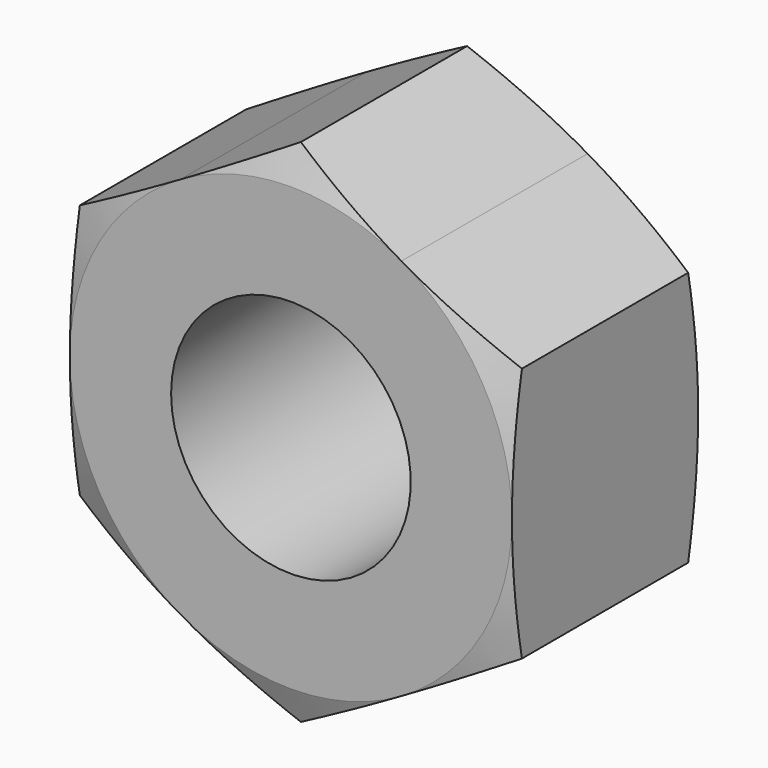
from build123d import *

# Parameters (mm, degrees)
F3_DEPTH      = 38
F3_DEPTH_BACK = 10.001
F4_D          = 10.3


# Not quite as in the source:
# - an extrude ends at something that could not be found from the text; its depth is read off the source's solid


with BuildPart() as f2:
    # F1 (on Right) → F2 (revolve)
    with BuildSketch(Plane.YZ):
        Polygon((-10, 0), (0, 0), (0, 9.5), (-0.5349107164, 10.9696551146), (-9.4650892836, 10.9696551146), (-10, 9.5), align=None)
    revolve(axis=Axis((0, -5, 0), (0, -1, 0)))

    # F0 (on Front) → F3 (cut, two sides)
    with BuildSketch(Plane.XZ) as f3_sk:
        with BuildLine():
            Line((-9.5, 5.4848275573), (-4.7499997575, 8.227241476))
            Line((-4.7499997575, 8.227241476), (0, 10.9696551146))
            ThreePointArc((0, 10.9696551146), (-5.4848275573, 9.5), (-9.5, 5.4848275573))
        make_face()
        with BuildLine():
            Line((-9.5, -5.4848275573), (-9.5, 0))
            Line((-9.5, 0), (-9.5, 5.4848275573))
            ThreePointArc((-9.5, 5.4848275573), (-10.9696551146, 0), (-9.5, -5.4848275573))
        make_face()
        with BuildLine():
            Line((0, 10.9696551146), (4.7500001405, 8.2272412548))
            Line((4.7500001405, 8.2272412548), (9.5, 5.4848275573))
            ThreePointArc((9.5, 5.4848275573), (5.4848275573, 9.5), (0, 10.9696551146))
        make_face()
        with BuildLine():
            Line((9.5, 5.4848275573), (9.5, 0))
            Line((9.5, 0), (9.5, -5.4848275573))
            ThreePointArc((9.5, -5.4848275573), (10.5958731807, -2.8391556619), (10.9696551146, 0))
            ThreePointArc((10.9696551146, 0), (10.5958731807, 2.8391556619), (9.5, 5.4848275573))
        make_face()
        with BuildLine():
            Line((9.5, -5.4848275573), (4.7500001405, -8.2272412548))
            Line((4.7500001405, -8.2272412548), (0, -10.9696551146))
            ThreePointArc((0, -10.9696551146), (5.4848275573, -9.5), (9.5, -5.4848275573))
        make_face()
        with BuildLine():
            Line((0, -10.9696551146), (-4.7499999942, -8.2272413393))
            Line((-4.7499999942, -8.2272413393), (-9.5, -5.4848275573))
            ThreePointArc((-9.5, -5.4848275573), (-5.4848275573, -9.5), (0, -10.9696551146))
        make_face()
    extrude(amount=-F3_DEPTH, mode=Mode.SUBTRACT)
    extrude(f3_sk.sketch, amount=F3_DEPTH_BACK, mode=Mode.SUBTRACT)

    # F4 (through all)
    with Locations(Plane(origin=(0, 0, 0), x_dir=(1, 0, 0), z_dir=(0, 1, 0))):
        with Locations((0, 0)):
            Hole(F4_D / 2)


solid = f2.part
